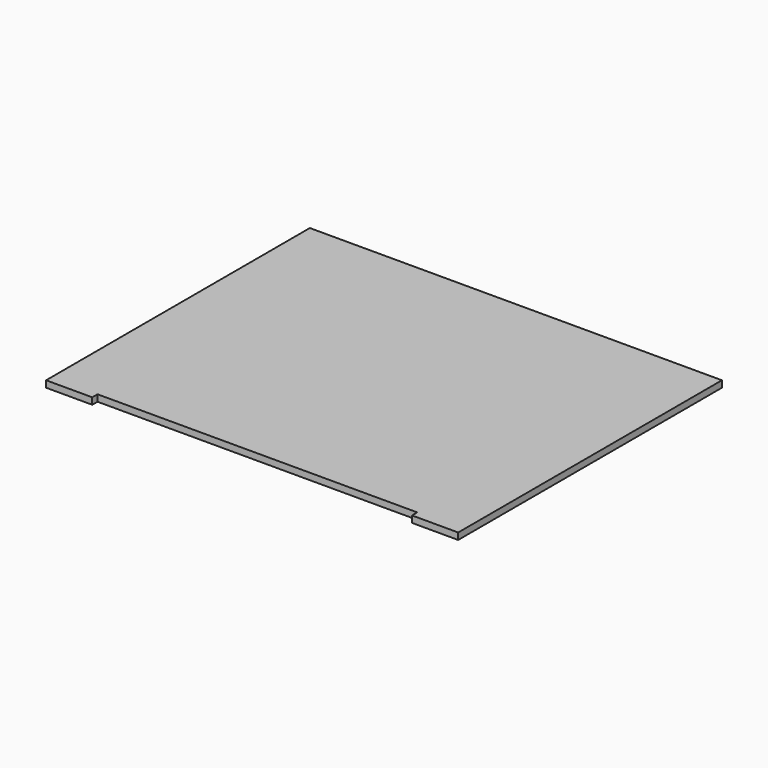
from build123d import *

# Parameters (mm, degrees)
F1_DEPTH = 8


# Not quite as in the source:
# - a feature names something its author has since deleted; it is built from what else it names


with BuildPart() as f1:
    # F0 (on Top) → F1 (new body)
    with BuildSketch(Plane.XY):
        Polygon((250, -200), (250, 200), (-250, 200), (-250, -200), (-194, -200), (-194, -192), (194, -192), (194, -200), align=None)
    extrude(amount=F1_DEPTH)


solid = f1.part
